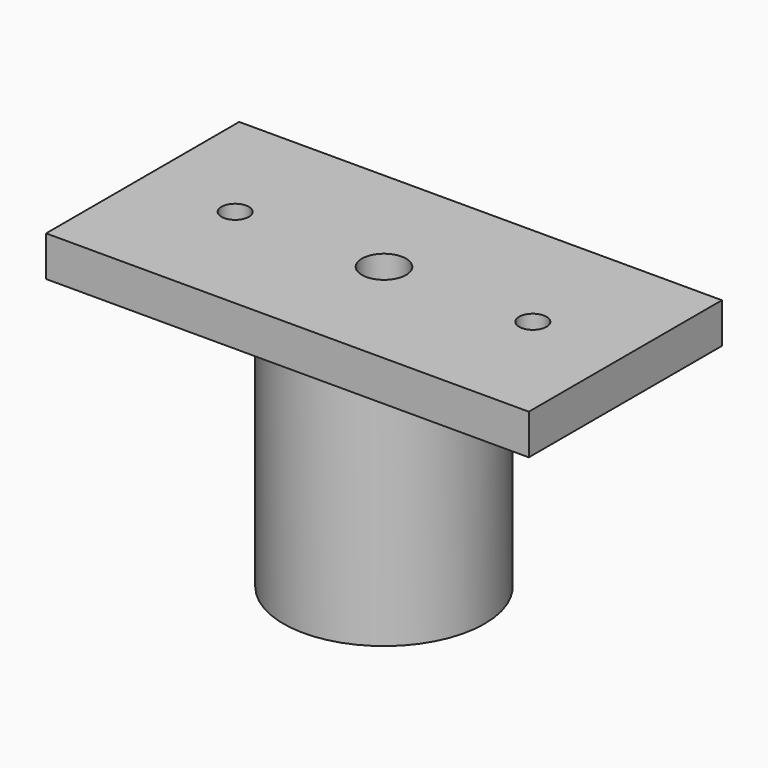
from build123d import *

# Parameters (mm, degrees)
F0_W     = 60
F0_H     = 30
F1_DEPTH = 35
F2_DEPTH = 30
F4_W     = 60
F4_H     = 30
F4_R     = 12.5
F5_DEPTH = 30
F7_D     = 3.4
F8_D     = 5.5


with BuildPart() as f1:
    # F0 (on Top) → F1 (new body)
    with BuildSketch(Plane.XY):
        Rectangle(F0_W, F0_H)
        with BuildLine():
            ThreePointArc((-2.5, -6.5383484153), (-3.9686269666, 5.7662812973), (7, 0))
            ThreePointArc((7, 0), (5.7662812973, -3.9686269666), (2.5, -6.5383484153))
            Line((2.5, -6.5383484153), (2.5, -9.5))
            Line((2.5, -9.5), (0, -9.5))
            Line((0, -9.5), (-2.5, -9.5))
            Line((-2.5, -9.5), (-2.5, -6.5383484153))
        make_face(mode=Mode.SUBTRACT)
        with BuildLine():
            ThreePointArc((2.5, -6.5383484153), (5.7662812973, -3.9686269666), (7, 0))
            ThreePointArc((7, 0), (-3.9686269666, 5.7662812973), (-2.5, -6.5383484153))
            ThreePointArc((-2.5, -6.5383484153), (0, -7), (2.5, -6.5383484153))
        make_face()
        with BuildLine():
            ThreePointArc((2.5, -6.5383484153), (0, -7), (-2.5, -6.5383484153))
            Line((-2.5, -6.5383484153), (-2.5, -9.5))
            Line((-2.5, -9.5), (0, -9.5))
            Line((0, -9.5), (2.5, -9.5))
            Line((2.5, -9.5), (2.5, -6.5383484153))
        make_face()
    extrude(amount=F1_DEPTH)

    # F0 (on Top) → F2 (cut)
    with BuildSketch(Plane.XY):
        with BuildLine():
            ThreePointArc((2.5, -6.5383484153), (5.7662812973, -3.9686269666), (7, 0))
            ThreePointArc((7, 0), (-3.9686269666, 5.7662812973), (-2.5, -6.5383484153))
            ThreePointArc((-2.5, -6.5383484153), (0, -7), (2.5, -6.5383484153))
        make_face()
        with BuildLine():
            ThreePointArc((2.5, -6.5383484153), (0, -7), (-2.5, -6.5383484153))
            Line((-2.5, -6.5383484153), (-2.5, -9.5))
            Line((-2.5, -9.5), (0, -9.5))
            Line((0, -9.5), (2.5, -9.5))
            Line((2.5, -9.5), (2.5, -6.5383484153))
        make_face()
    extrude(amount=F2_DEPTH, mode=Mode.SUBTRACT)

    # F4 (on face) → F5 (cut)
    with BuildSketch(Plane.XY):
        Rectangle(F4_W, F4_H)
        Circle(F4_R, mode=Mode.SUBTRACT)
    extrude(amount=F5_DEPTH, mode=Mode.SUBTRACT)

    # F7 (through all)
    with Locations(Plane.XY.offset(35)):
        with Locations((-18.5, 0), (18.5, 0)):
            Hole(F7_D / 2)

    # F8 (through all)
    with Locations(Plane(origin=(0, 0, 0), x_dir=(1, 0, 0), z_dir=(0, 0, -1))):
        with Locations((0, 0)):
            Hole(F8_D / 2)


solid = f1.part
